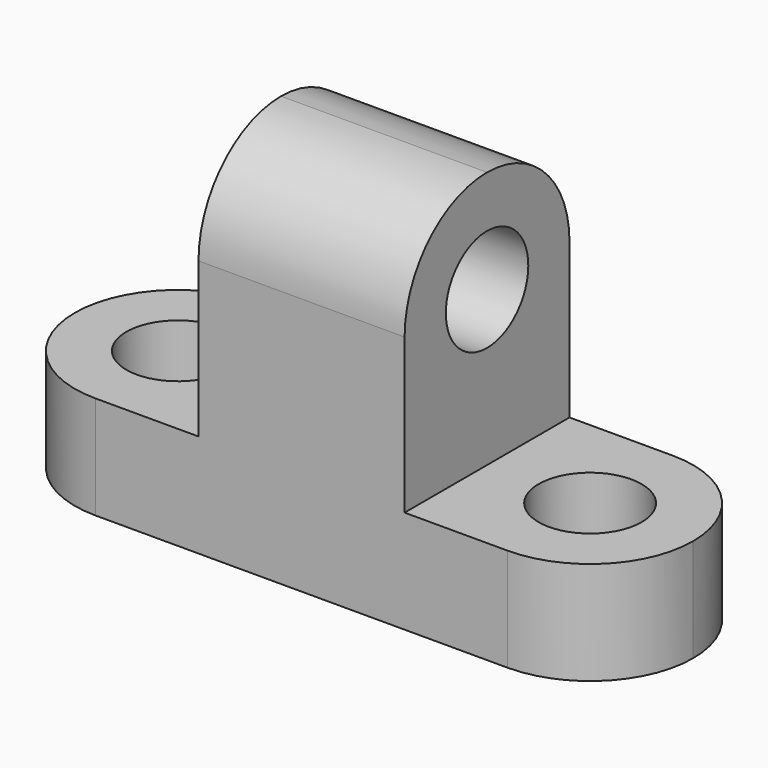
from build123d import *

# Parameters (mm, degrees)
F1_DEPTH = 25.4
F2_R     = 12.69999
F3_R     = 6.35
F4_DEPTH = 25.4
F5_R     = 6.35
F6_DEPTH = 25.4
F7_R     = 6.35
F8_DEPTH = 25.4


# Not quite as in the source:
# - a fillet or chamfer is up to 0.001 mm smaller than in the source, because OpenCascade refuses the exact size


with BuildPart() as f1:
    # F0 (on Front) → F1 (new body)
    with BuildSketch(Plane.XZ):
        Polygon((0, 12.7), (0, 0), (76.2, 0), (76.2, 12.7), (50.8, 12.7), (50.8, 44.45), (25.4, 44.45), (25.4, 12.7), align=None)
    extrude(amount=F1_DEPTH)

    # F2 (radius 12.7 in the source; OpenCascade refuses exactly that, so slightly less here)
    f2_edges = [f1.edges().sort_by_distance(p)[0] for p in [
        (38.1, -25.4, 44.45),
        (38.1, 0, 44.45),
        (0, -25.4, 6.35),
        (76.2, -25.4, 6.35),
        (76.2, 0, 6.35),
        (0, 0, 6.35),
    ]]
    fillet(f2_edges, radius=F2_R)

    # F3 (on face) → F4 (cut)
    with BuildSketch(Plane.YZ.offset(50.8)):
        with Locations((-12.7, 31.75)):
            Circle(F3_R)
    extrude(amount=-F4_DEPTH, mode=Mode.SUBTRACT)

    # F5 (on face) → F6 (cut)
    with BuildSketch(Plane.XY.offset(12.7)):
        with Locations((12.7, -12.7)):
            Circle(F5_R)
    extrude(amount=-F6_DEPTH, mode=Mode.SUBTRACT)

    # F7 (on face) → F8 (cut)
    with BuildSketch(Plane.XY.offset(12.7)):
        with Locations((63.5, -12.7)):
            Circle(F7_R)
    extrude(amount=-F8_DEPTH, mode=Mode.SUBTRACT)


solid = f1.part
